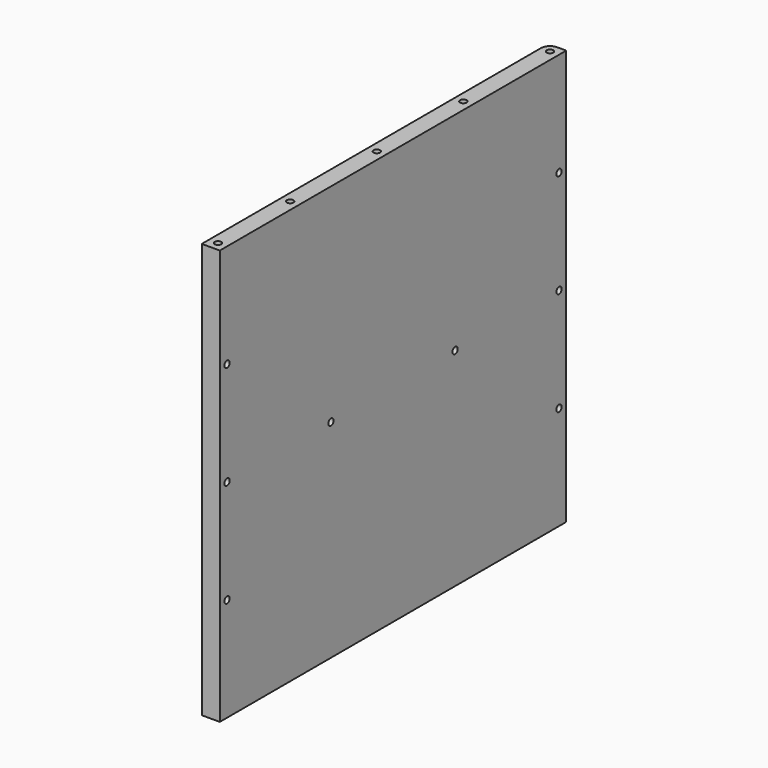
from build123d import *

# Parameters (mm, degrees)
F0_W           = 18
F0_H           = 414
F1_DEPTH       = 432
F2_R           = 9
F6_D           = 6.6
F6_DEPTH       = 5
F6_TIP         = 1.9828400428
F6_ON_F3_D     = 6.6
F6_ON_F3_DEPTH = 5
F6_ON_F3_TIP   = 1.9828400428
F6_ON_F5_D     = 6.6
F6_ON_F5_DEPTH = 5
F6_ON_F5_TIP   = 1.9828400428
F7_ANGLE       = 180


# Not quite as in the source:
# - a feature names something its author has since deleted; it is built from what else it names


with BuildPart() as f1:
    # F0 (on Front) → F1 (new body)
    with BuildSketch(Plane.XZ):
        with Locations((9, -7.566531274)):
            Rectangle(F0_W, F0_H)
    extrude(amount=F1_DEPTH)

    # F2
    f2_edges = [f1.edges().sort_by_distance(p)[0] for p in [
        (18, 0, -7.566531),
    ]]
    fillet(f2_edges, radius=F2_R)

    # F6
    with Locations(Plane(origin=(0, 0, -214.566531274), x_dir=(1, 0, 0), z_dir=(0, 0, -1))):
        with Locations((9, 9), (9, 117), (9, 225), (9, 333), (9, 423)):
            Hole(F6_D / 2, depth=F6_DEPTH)
            with Locations((0, 0, -(F6_DEPTH + F6_TIP / 2))):  # 118° drill point
                Cone(0, F6_D / 2, F6_TIP, mode=Mode.SUBTRACT)

    # F6 on F3
    with Locations(Plane(origin=(0, 0, 0), x_dir=(0, -1, 0), z_dir=(-1, 0, 0))):
        with Locations((423, -111.066531274), (423, -7.566531274), (423, 95.933468726), (9, -111.066531274), (9, -7.566531274), (9, 95.933468726), (138.6, -7.566531274), (293.4, -7.566531274)):
            Hole(F6_ON_F3_D / 2, depth=F6_ON_F3_DEPTH)
            with Locations((0, 0, -(F6_ON_F3_DEPTH + F6_ON_F3_TIP / 2))):  # 118° drill point
                Cone(0, F6_ON_F3_D / 2, F6_ON_F3_TIP, mode=Mode.SUBTRACT)

    # F6 on F5
    with Locations(Plane.XY.offset(199.433468726)):
        with Locations((9, -117), (9, -225), (9, -333), (9, -9), (9, -423)):
            Hole(F6_ON_F5_D / 2, depth=F6_ON_F5_DEPTH)
            with Locations((0, 0, -(F6_ON_F5_DEPTH + F6_ON_F5_TIP / 2))):  # 118° drill point
                Cone(0, F6_ON_F5_D / 2, F6_ON_F5_TIP, mode=Mode.SUBTRACT)


with BuildPart() as f1_1:
    # F7: moved
    add(f1.part.rotate(Axis((0, -216, 199.433468726), (0, 1, 0)), F7_ANGLE))


solid = f1_1.part
